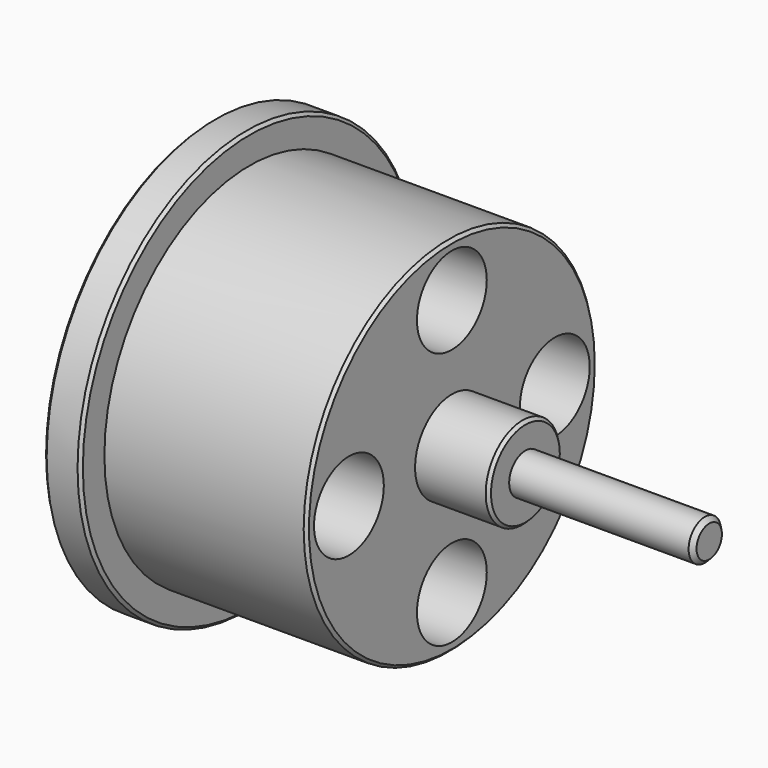
from build123d import *

# Parameters (mm, degrees)
F0_R            = 73.025
F1_DEPTH        = 12.7
F2_R            = 62.70625
F3_DEPTH        = 69.85
F4_R            = 15.875
F5_DEPTH        = 25.4
F6_R            = 7
F7_DEPTH        = 63.5
F8_SIZE         = 1.016
F9_SIZE         = 1.524
F11_D           = 20.6375
F11_CBORE_D     = 30.1498
F11_CBORE_DEPTH = 50.8


# Not quite as in the source:
# - a length typed as a fraction of an inch, garbled in the dataset ("3 / 203.2 mm" for 3/8 in), is restored


with BuildPart() as f1:
    # F0 (on Right) → F1 (new body)
    with BuildSketch(Plane.YZ):
        Circle(F0_R)
    extrude(amount=F1_DEPTH)

    # F2 (on face) → F3 (join)
    with BuildSketch(Plane.YZ.offset(12.7)):
        Circle(F2_R)
    extrude(amount=F3_DEPTH)

    # F4 (on face) → F5 (join)
    with BuildSketch(Plane.YZ.offset(82.55)):
        Circle(F4_R)
    extrude(amount=F5_DEPTH)

    # F6 (on face) → F7 (join)
    with BuildSketch(Plane.YZ.offset(107.95)):
        Circle(F6_R)
    extrude(amount=F7_DEPTH)

    # F8
    f8_edges = [f1.edges().sort_by_distance(p)[0] for p in [
        (6.35, 73.025, 0),
        (0, -73.025, 0),
        (12.7, -73.025, 0),
        (82.55, -62.70625, 0),
        (107.95, -15.875, 0),
    ]]
    chamfer(f8_edges, length=F8_SIZE)

    # F9
    f9_edges = [f1.edges().sort_by_distance(p)[0] for p in [
        (171.45, -7, 0),
    ]]
    chamfer(f9_edges, length=F9_SIZE)

    # F11 (through all)
    with Locations(Plane.YZ.offset(82.55)):
        with Locations((0, 44.45), (44.45, 0), (0, -44.45), (-44.45, 0)):
            CounterBoreHole(F11_D / 2, F11_CBORE_D / 2, F11_CBORE_DEPTH)


solid = f1.part
